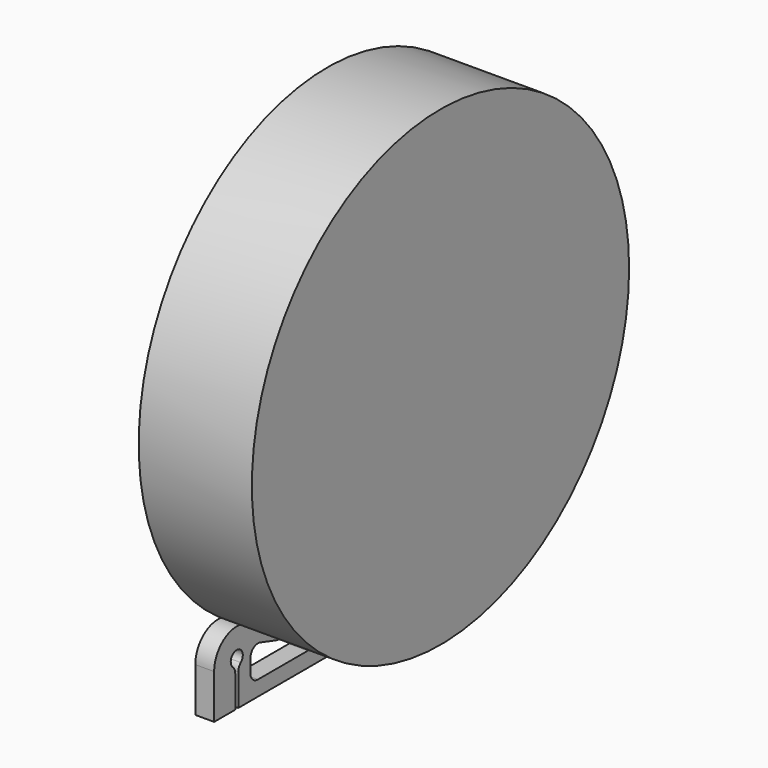
from build123d import *

# Parameters (mm, degrees)
F0_R        = 125
F1_DEPTH    = 60
F3_DEPTH    = 10
F4_T1_DEPTH = 10
F4_T3_DEPTH = 24.1761029315


# Not quite as in the source:
# - a fillet or chamfer that OpenCascade refuses, or shapes differently, is made with other operations: its cross-section is extruded or revolved along the edge and cut away or added
# - a feature names something its author has since deleted; it is built from what else it names


with BuildPart() as f1:
    # F0 (on Right) → F1 (new body)
    with BuildSketch(Plane.YZ):
        Circle(F0_R)
    extrude(amount=F1_DEPTH)


with BuildPart() as f3:
    # F2 (on face) → F3 (new body)
    with BuildSketch(Plane(origin=(0, 0, 0), x_dir=(0, -1, 0), z_dir=(-1, 0, 0))):
        with BuildLine():
            ThreePointArc((0, -125), (-27.4562289572, -121.9473472096), (-53.5714285714, -112.9384878632))
            ThreePointArc((-53.5714285714, -112.9384878632), (-68.0178372574, -113.8137925858), (-75, -126.4911064067))
            Line((-75, -126.4911064067), (-75, -150))
            Line((-75, -150), (-61, -150))
            Line((-61, -150), (-61, -130.3640897529))
            ThreePointArc((-61, -130.3640897529), (-60, -122.4911064067), (-59, -130.3640897529))
            Line((-59, -130.3640897529), (-59, -150))
            Line((-59, -150), (0, -150))
            Line((0, -150), (0, -125))
        make_face()
        with BuildLine():
            Line((-8.00000038, -141.99999962), (-50.99999962, -141.99999962))
            Line((-50.99999962, -141.99999962), (-50.99999962, -130.3640897529))
            Line((-50.99999962, -130.3640897529), (-50.99999962, -122.8332208315))
            ThreePointArc((-50.99999962, -122.8332208315), (-29.914564521, -129.5921252646), (-8.00000038, -132.7591808313))
            Line((-8.00000038, -132.7591808313), (-8.00000038, -141.99999962))
        make_face(mode=Mode.SUBTRACT)
    extrude(amount=F3_DEPTH)

    # F4: fillet of radius 5 on 6 edges, made by hand

    # F4_s2 → F4_t1 (join)
    with BuildSketch(Plane.YZ.offset(-10)):
        with BuildLine():
            ThreePointArc((44.3333329717, -125.3936030613), (48.8867509739, -126.0251653767), (50.99999962, -130.1076482757))
            Line((50.99999962, -130.1076482757), (50.99999962, -122.8332208315))
            ThreePointArc((50.99999962, -122.8332208315), (47.6838543435, -124.1581658048), (44.3333329717, -125.3936030613))
        make_face()
        with BuildLine():
            ThreePointArc((50.99999962, -136.99999962), (49.535533526, -140.535533526), (45.99999962, -141.99999962))
            Line((45.99999962, -141.99999962), (50.99999962, -141.99999962))
            Line((50.99999962, -141.99999962), (50.99999962, -136.99999962))
        make_face()
        with BuildLine():
            ThreePointArc((13.00000038, -141.99999962), (9.464466474, -140.535533526), (8.00000038, -136.99999962))
            Line((8.00000038, -136.99999962), (8.00000038, -141.99999962))
            Line((8.00000038, -141.99999962), (13.00000038, -141.99999962))
        make_face()
        with BuildLine():
            ThreePointArc((12.5289858748, -132.4085518916), (9.3016850523, -134.0214301028), (8.00000038, -137.3863169861))
            Line((8.00000038, -137.3863169861), (8.00000038, -132.7591808313))
            ThreePointArc((8.00000038, -132.7591808313), (10.2659901775, -132.6032033804), (12.5289858748, -132.4085518916))
        make_face()
    extrude(amount=F4_T1_DEPTH)

    # F4_s4 → F4_t3 (cut)
    with BuildSketch(Plane.YZ.offset(-17.0880514658)):
        with BuildLine():
            ThreePointArc((57.3333333333, -129.4725303767), (58.5643546459, -131.1580688869), (59, -133.1993103392))
            Line((59, -133.1993103392), (59, -130.3640897529))
            ThreePointArc((59, -130.3640897529), (58.1132486541, -130.018168833), (57.3333333333, -129.4725303767))
        make_face()
        with BuildLine():
            ThreePointArc((61, -133.1993103392), (61.4356453541, -131.1580688869), (62.6666666667, -129.4725303767))
            ThreePointArc((62.6666666667, -129.4725303767), (61.8867513459, -130.018168833), (61, -130.3640897529))
            Line((61, -130.3640897529), (61, -133.1993103392))
        make_face()
    extrude(amount=F4_T3_DEPTH, mode=Mode.SUBTRACT)

    # F5: F3 across face


with BuildPart() as f3_1:
    add(f3.part)
    add(f3.part.mirror(Plane(origin=(-5, 0, -137.5), x_dir=(1, 0, 0), z_dir=(0, -1, 0))))


solid = Compound([f1.part, f3_1.part])
